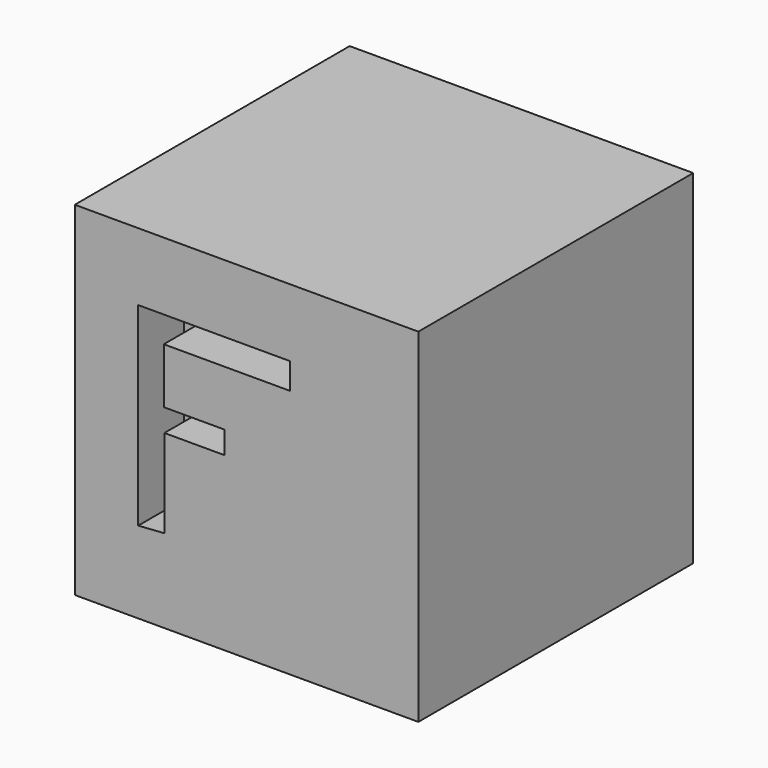
from build123d import *

# Parameters (mm, degrees)
F1_W     = 152.4
F1_H     = 152.4
F2_DEPTH = 76.2
F4_DEPTH = 25.4
F6_DEPTH = 25.4


# Not quite as in the source:
# - a variable given as a bare number and used for a length is read in inches; the dataset says mm whatever the document's units were


with BuildPart() as f2:
    # F1 (on Front) → F2 (new body, symmetric)
    with BuildSketch(Plane.XZ):
        Rectangle(F1_W, F1_H)
    extrude(amount=F2_DEPTH, both=True)

    # F3 (on face) → F4 (cut)
    with BuildSketch(Plane.XZ.offset(76.2)):
        Polygon((19.1713254899, 46.1731813848), (-48.0633080006, 46.1731813848), (-48.0633080006, -39.9627536535), (-36.4525094628, -39.1526967287), (-36.4525094628, 0), (-9.720666334, 0), (-9.720666334, 9.9906884134), (-36.7225259542, 9.9906884134), (-36.7225259542, 34.5623828471), (19.1713254899, 34.5623828471), align=None)
    extrude(amount=-F4_DEPTH, mode=Mode.SUBTRACT)

    # F5 (on face) → F6 (join)
    with BuildSketch(Plane(origin=(0, 76.2, 0), x_dir=(-1, 0, 0), z_dir=(0, 1, 0))):
        Polygon((48.0633080006, -39.9627536535), (48.0633080006, 46.1731813848), (-19.1713254899, 46.1731813848), (-19.1713254899, 34.5623828471), (36.7225259542, 34.5623828471), (36.7225259542, 9.9906884134), (9.720666334, 9.9906884134), (9.720666334, 0), (36.4525094628, 0), (36.4525094628, -39.1526967287), align=None)
    extrude(amount=F6_DEPTH)


solid = f2.part
